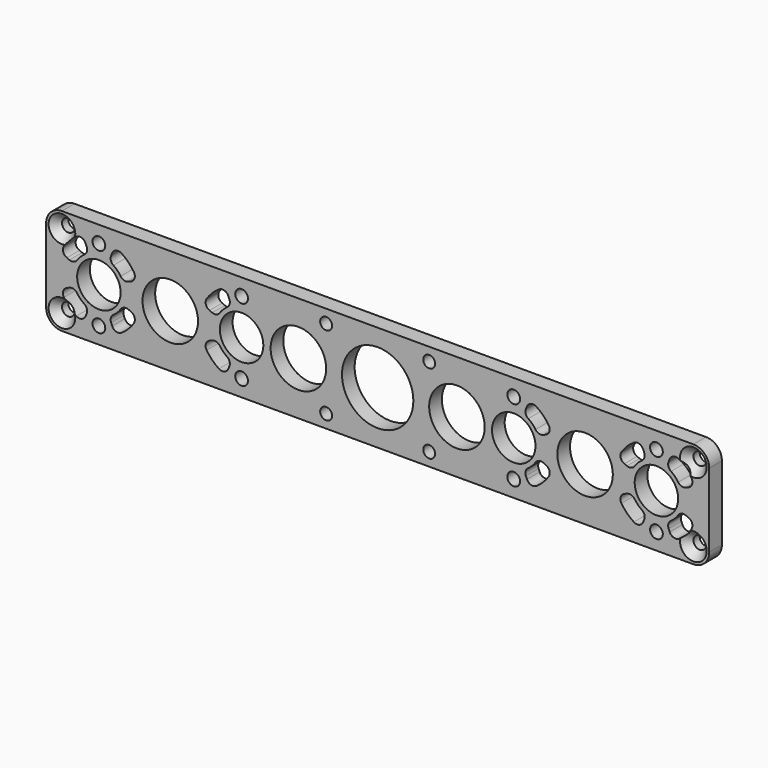
from build123d import *

# Parameters (mm, degrees)
F0_R      = 2.5527
F0_R_2    = 8.6995
F0_R_3    = 11.1125
F0_R_4    = 14.2875
F1_DEPTH  = 6.35
F2_R      = 2.38125
F3_DEPTH  = 6.351
F15_DEPTH = 25.4


with BuildPart() as f1:
    # F0 (on Front) → F1 (new body)
    with BuildSketch(Plane.XZ):
        with BuildLine():
            Line((111.633, 21.1455), (-111.633, 21.1455))
            Line((-111.633, 21.1455), (-126.4285, 21.1455))
            ThreePointArc((-126.4285, 21.1455), (-130.9186280605, 19.2856280605), (-132.7785, 14.7955))
            Line((-132.7785, 14.7955), (-132.7785, -14.7955))
            ThreePointArc((-132.7785, -14.7955), (-130.9186280605, -19.2856280605), (-126.4285, -21.1455))
            Line((-126.4285, -21.1455), (-111.633, -21.1455))
            Line((-111.633, -21.1455), (111.633, -21.1455))
            Line((111.633, -21.1455), (126.4285, -21.1455))
            ThreePointArc((126.4285, -21.1455), (130.9186280605, -19.2856280605), (132.7785, -14.7955))
            Line((132.7785, -14.7955), (132.7785, 14.7955))
            ThreePointArc((132.7785, 14.7955), (130.9186280605, 19.2856280605), (126.4285, 21.1455))
            Line((126.4285, 21.1455), (111.633, 21.1455))
        make_face()
        with Locations((-126.4285, -14.7955)):
            Circle(F0_R, mode=Mode.SUBTRACT)
        with Locations((-111.633, -14.5)):
            Circle(F0_R, mode=Mode.SUBTRACT)
        with Locations((-54.483, -14.5)):
            Circle(F0_R, mode=Mode.SUBTRACT)
        with Locations((54.483, -14.5)):
            Circle(F0_R, mode=Mode.SUBTRACT)
        with Locations((111.633, -14.5)):
            Circle(F0_R, mode=Mode.SUBTRACT)
        with Locations((126.4285, -14.7955)):
            Circle(F0_R, mode=Mode.SUBTRACT)
        with Locations((-111.633, 0)):
            Circle(F0_R_2, mode=Mode.SUBTRACT)
        with Locations((-83.058, 0)):
            Circle(F0_R_3, mode=Mode.SUBTRACT)
        with Locations((-54.483, 0)):
            Circle(F0_R_2, mode=Mode.SUBTRACT)
        with Locations((-31.75, 0)):
            Circle(F0_R_3, mode=Mode.SUBTRACT)
        with Locations((-126.4285, 14.7955)):
            Circle(F0_R, mode=Mode.SUBTRACT)
        with Locations((-111.633, 14.5)):
            Circle(F0_R, mode=Mode.SUBTRACT)
        with Locations((-54.483, 14.5)):
            Circle(F0_R, mode=Mode.SUBTRACT)
        Circle(F0_R_4, mode=Mode.SUBTRACT)
        with Locations((31.75, 0)):
            Circle(F0_R_3, mode=Mode.SUBTRACT)
        with Locations((54.483, 0)):
            Circle(F0_R_2, mode=Mode.SUBTRACT)
        with Locations((83.058, 0)):
            Circle(F0_R_3, mode=Mode.SUBTRACT)
        with Locations((111.633, 0)):
            Circle(F0_R_2, mode=Mode.SUBTRACT)
        with Locations((54.483, 14.5)):
            Circle(F0_R, mode=Mode.SUBTRACT)
        with Locations((111.633, 14.5)):
            Circle(F0_R, mode=Mode.SUBTRACT)
        with Locations((126.4285, 14.7955)):
            Circle(F0_R, mode=Mode.SUBTRACT)
    extrude(amount=F1_DEPTH)

    # F2 (on face) → F3 (cut, through all)
    with BuildSketch(Plane.XZ.offset(6.35)):
        with Locations((20.6375, 15.875)):
            Circle(F2_R)
        with Locations((20.6375, -15.875)):
            Circle(F2_R)
        with Locations((-20.6375, -15.875)):
            Circle(F2_R)
        with Locations((-20.6375, 15.875)):
            Circle(F2_R)
    extrude(amount=-F3_DEPTH, mode=Mode.SUBTRACT)

    # F5 (on offset) → F6 (revolve, cut)
    with BuildSketch(Plane.YZ.offset(126.4285)):
        Polygon((-6.35, 20.1396451588), (-6.35, 14.7955), (-3.1242, 14.7955), (-3.1242, 17.3355), align=None)
    revolve(axis=Axis((126.4285, -4.7371, 14.7955), (0, 1, 0)), mode=Mode.SUBTRACT)

    # F7 (on offset) → F8 (revolve, cut)
    with BuildSketch(Plane.YZ.offset(126.4285)):
        Polygon((-6.35, -9.4513548412), (-6.35, -14.7955), (-3.1242, -14.7955), (-3.1242, -12.2555), align=None)
    revolve(axis=Axis((126.4285, -4.7371, -14.7955), (0, 1, 0)), mode=Mode.SUBTRACT)

    # F10 (on offset) → F11 (revolve, cut)
    with BuildSketch(Plane(origin=(-126.4285, 0, 0), x_dir=(0, -1, 0), z_dir=(-1, 0, 0))):
        Polygon((6.35, 9.4513548412), (6.35, 14.7955), (3.1242, 14.7955), (3.1242, 12.2555), align=None)
    revolve(axis=Axis((-126.4285, -4.7371, 14.7955), (0, 1, 0)), mode=Mode.SUBTRACT)

    # F12 (on offset) → F13 (revolve, cut)
    with BuildSketch(Plane(origin=(-126.4285, 0, 0), x_dir=(0, -1, 0), z_dir=(-1, 0, 0))):
        Polygon((6.35, -20.1396451588), (6.35, -14.7955), (3.1242, -14.7955), (3.1242, -17.3355), align=None)
    revolve(axis=Axis((-126.4285, -4.7371, -14.7955), (0, 1, 0)), mode=Mode.SUBTRACT)

    # F14 (on face) → F15 (cut)
    with BuildSketch(Plane(origin=(0, 0, 0), x_dir=(-1, 0, 0), z_dir=(0, 1, 0))):
        with BuildLine():
            Line((106.3142512649, -12.840595331), (106.7471694564, -11.7954383619))
            ThreePointArc((106.7471694564, -11.7954383619), (106.8311557852, -10.0861385562), (105.8117319426, -8.7115351376))
            ThreePointArc((105.8117319426, -8.7115351376), (104.2242887001, -7.4087112999), (102.9214648624, -5.8212680574))
            ThreePointArc((102.9214648624, -5.8212680574), (101.5468614438, -4.8018442148), (99.8375616381, -4.8858305436))
            Line((99.8375616381, -4.8858305436), (98.792404669, -5.3187487351))
            ThreePointArc((98.792404669, -5.3187487351), (97.3396139347, -6.9091536496), (97.6307433893, -9.0434526798))
            ThreePointArc((97.6307433893, -9.0434526798), (99.8464138411, -11.7865861589), (102.5895473202, -14.0022566107))
            ThreePointArc((102.5895473202, -14.0022566107), (104.7238463504, -14.2933860653), (106.3142512649, -12.840595331))
        make_face()
        with BuildLine():
            Line((98.792404669, 5.3187487351), (99.8375616381, 4.8858305436))
            ThreePointArc((99.8375616381, 4.8858305436), (101.5468614438, 4.8018442148), (102.9214648624, 5.8212680574))
            ThreePointArc((102.9214648624, 5.8212680574), (104.2242887001, 7.4087112999), (105.8117319426, 8.7115351376))
            ThreePointArc((105.8117319426, 8.7115351376), (106.8311557852, 10.0861385562), (106.7471694564, 11.7954383619))
            Line((106.7471694564, 11.7954383619), (106.3142512649, 12.840595331))
            ThreePointArc((106.3142512649, 12.840595331), (104.7238463504, 14.2933860653), (102.5895473202, 14.0022566107))
            ThreePointArc((102.5895473202, 14.0022566107), (99.8464138411, 11.7865861589), (97.6307433893, 9.0434526798))
            ThreePointArc((97.6307433893, 9.0434526798), (97.3396139347, 6.9091536496), (98.792404669, 5.3187487351))
        make_face()
        with BuildLine():
            Line((116.9517487351, 12.840595331), (116.5188305436, 11.7954383619))
            ThreePointArc((116.5188305436, 11.7954383619), (116.4348442148, 10.0861385562), (117.4542680574, 8.7115351376))
            ThreePointArc((117.4542680574, 8.7115351376), (119.0417112999, 7.4087112999), (120.3445351376, 5.8212680574))
            ThreePointArc((120.3445351376, 5.8212680574), (121.7191385562, 4.8018442148), (123.4284383619, 4.8858305436))
            Line((123.4284383619, 4.8858305436), (124.473595331, 5.3187487351))
            ThreePointArc((124.473595331, 5.3187487351), (125.9263860653, 6.9091536496), (125.6352566107, 9.0434526798))
            ThreePointArc((125.6352566107, 9.0434526798), (123.4195861589, 11.7865861589), (120.6764526798, 14.0022566107))
            ThreePointArc((120.6764526798, 14.0022566107), (118.5421536496, 14.2933860653), (116.9517487351, 12.840595331))
        make_face()
        with BuildLine():
            Line((124.473595331, -5.3187487351), (123.4284383619, -4.8858305436))
            ThreePointArc((123.4284383619, -4.8858305436), (121.7191385562, -4.8018442148), (120.3445351376, -5.8212680574))
            ThreePointArc((120.3445351376, -5.8212680574), (119.0417112999, -7.4087112999), (117.4542680574, -8.7115351376))
            ThreePointArc((117.4542680574, -8.7115351376), (116.4348442148, -10.0861385562), (116.5188305436, -11.7954383619))
            Line((116.5188305436, -11.7954383619), (116.9517487351, -12.840595331))
            ThreePointArc((116.9517487351, -12.840595331), (118.5421536496, -14.2933860653), (120.6764526798, -14.0022566107))
            ThreePointArc((120.6764526798, -14.0022566107), (123.4195861589, -11.7865861589), (125.6352566107, -9.0434526798))
            ThreePointArc((125.6352566107, -9.0434526798), (125.9263860653, -6.9091536496), (124.473595331, -5.3187487351))
        make_face()
        with BuildLine():
            Line((59.8017487351, 12.840595331), (59.3688305436, 11.7954383619))
            ThreePointArc((59.3688305436, 11.7954383619), (59.2848442148, 10.0861385562), (60.3042680574, 8.7115351376))
            ThreePointArc((60.3042680574, 8.7115351376), (61.8917112999, 7.4087112999), (63.1945351376, 5.8212680574))
            ThreePointArc((63.1945351376, 5.8212680574), (64.5691385562, 4.8018442148), (66.2784383619, 4.8858305436))
            Line((66.2784383619, 4.8858305436), (67.323595331, 5.3187487351))
            ThreePointArc((67.323595331, 5.3187487351), (68.7763860653, 6.9091536496), (68.4852566107, 9.0434526798))
            ThreePointArc((68.4852566107, 9.0434526798), (66.2695861589, 11.7865861589), (63.5264526798, 14.0022566107))
            ThreePointArc((63.5264526798, 14.0022566107), (61.3921536496, 14.2933860653), (59.8017487351, 12.840595331))
        make_face()
        with BuildLine():
            Line((67.323595331, -5.3187487351), (66.2784383619, -4.8858305436))
            ThreePointArc((66.2784383619, -4.8858305436), (64.5691385562, -4.8018442148), (63.1945351376, -5.8212680574))
            ThreePointArc((63.1945351376, -5.8212680574), (61.8917112999, -7.4087112999), (60.3042680574, -8.7115351376))
            ThreePointArc((60.3042680574, -8.7115351376), (59.2848442148, -10.0861385562), (59.3688305436, -11.7954383619))
            Line((59.3688305436, -11.7954383619), (59.8017487351, -12.840595331))
            ThreePointArc((59.8017487351, -12.840595331), (61.3921536496, -14.2933860653), (63.5264526798, -14.0022566107))
            ThreePointArc((63.5264526798, -14.0022566107), (66.2695861589, -11.7865861589), (68.4852566107, -9.0434526798))
            ThreePointArc((68.4852566107, -9.0434526798), (68.7763860653, -6.9091536496), (67.323595331, -5.3187487351))
        make_face()
        with BuildLine():
            Line((-59.8017487351, -12.840595331), (-59.3688305436, -11.7954383619))
            ThreePointArc((-59.3688305436, -11.7954383619), (-59.2848442148, -10.0861385562), (-60.3042680574, -8.7115351376))
            ThreePointArc((-60.3042680574, -8.7115351376), (-61.8917112999, -7.4087112999), (-63.1945351376, -5.8212680574))
            ThreePointArc((-63.1945351376, -5.8212680574), (-64.5691385562, -4.8018442148), (-66.2784383619, -4.8858305436))
            Line((-66.2784383619, -4.8858305436), (-67.323595331, -5.3187487351))
            ThreePointArc((-67.323595331, -5.3187487351), (-68.7763860653, -6.9091536496), (-68.4852566107, -9.0434526798))
            ThreePointArc((-68.4852566107, -9.0434526798), (-66.2695861589, -11.7865861589), (-63.5264526798, -14.0022566107))
            ThreePointArc((-63.5264526798, -14.0022566107), (-61.3921536496, -14.2933860653), (-59.8017487351, -12.840595331))
        make_face()
        with BuildLine():
            Line((-67.323595331, 5.3187487351), (-66.2784383619, 4.8858305436))
            ThreePointArc((-66.2784383619, 4.8858305436), (-64.5691385562, 4.8018442148), (-63.1945351376, 5.8212680574))
            ThreePointArc((-63.1945351376, 5.8212680574), (-61.8917112999, 7.4087112999), (-60.3042680574, 8.7115351376))
            ThreePointArc((-60.3042680574, 8.7115351376), (-59.2848442148, 10.0861385562), (-59.3688305436, 11.7954383619))
            Line((-59.3688305436, 11.7954383619), (-59.8017487351, 12.840595331))
            ThreePointArc((-59.8017487351, 12.840595331), (-61.3921536496, 14.2933860653), (-63.5264526798, 14.0022566107))
            ThreePointArc((-63.5264526798, 14.0022566107), (-66.2695861589, 11.7865861589), (-68.4852566107, 9.0434526798))
            ThreePointArc((-68.4852566107, 9.0434526798), (-68.7763860653, 6.9091536496), (-67.323595331, 5.3187487351))
        make_face()
        with BuildLine():
            Line((-116.9517487351, -12.840595331), (-116.5188305436, -11.7954383619))
            ThreePointArc((-116.5188305436, -11.7954383619), (-116.4348442148, -10.0861385562), (-117.4542680574, -8.7115351376))
            ThreePointArc((-117.4542680574, -8.7115351376), (-119.0417112999, -7.4087112999), (-120.3445351376, -5.8212680574))
            ThreePointArc((-120.3445351376, -5.8212680574), (-121.7191385562, -4.8018442148), (-123.4284383619, -4.8858305436))
            Line((-123.4284383619, -4.8858305436), (-124.473595331, -5.3187487351))
            ThreePointArc((-124.473595331, -5.3187487351), (-125.9263860653, -6.9091536496), (-125.6352566107, -9.0434526798))
            ThreePointArc((-125.6352566107, -9.0434526798), (-123.4195861589, -11.7865861589), (-120.6764526798, -14.0022566107))
            ThreePointArc((-120.6764526798, -14.0022566107), (-118.5421536496, -14.2933860653), (-116.9517487351, -12.840595331))
        make_face()
        with BuildLine():
            Line((-124.473595331, 5.3187487351), (-123.4284383619, 4.8858305436))
            ThreePointArc((-123.4284383619, 4.8858305436), (-121.7191385562, 4.8018442148), (-120.3445351376, 5.8212680574))
            ThreePointArc((-120.3445351376, 5.8212680574), (-119.0417112999, 7.4087112999), (-117.4542680574, 8.7115351376))
            ThreePointArc((-117.4542680574, 8.7115351376), (-116.4348442148, 10.0861385562), (-116.5188305436, 11.7954383619))
            Line((-116.5188305436, 11.7954383619), (-116.9517487351, 12.840595331))
            ThreePointArc((-116.9517487351, 12.840595331), (-118.5421536496, 14.2933860653), (-120.6764526798, 14.0022566107))
            ThreePointArc((-120.6764526798, 14.0022566107), (-123.4195861589, 11.7865861589), (-125.6352566107, 9.0434526798))
            ThreePointArc((-125.6352566107, 9.0434526798), (-125.9263860653, 6.9091536496), (-124.473595331, 5.3187487351))
        make_face()
        with BuildLine():
            Line((-106.3142512649, 12.840595331), (-106.7471694564, 11.7954383619))
            ThreePointArc((-106.7471694564, 11.7954383619), (-106.8311557852, 10.0861385562), (-105.8117319426, 8.7115351376))
            ThreePointArc((-105.8117319426, 8.7115351376), (-104.2242887001, 7.4087112999), (-102.9214648624, 5.8212680574))
            ThreePointArc((-102.9214648624, 5.8212680574), (-101.5468614438, 4.8018442148), (-99.8375616381, 4.8858305436))
            Line((-99.8375616381, 4.8858305436), (-98.792404669, 5.3187487351))
            ThreePointArc((-98.792404669, 5.3187487351), (-97.3396139347, 6.9091536496), (-97.6307433893, 9.0434526798))
            ThreePointArc((-97.6307433893, 9.0434526798), (-99.8464138411, 11.7865861589), (-102.5895473202, 14.0022566107))
            ThreePointArc((-102.5895473202, 14.0022566107), (-104.7238463504, 14.2933860653), (-106.3142512649, 12.840595331))
        make_face()
        with BuildLine():
            Line((-98.792404669, -5.3187487351), (-99.8375616381, -4.8858305436))
            ThreePointArc((-99.8375616381, -4.8858305436), (-101.5468614438, -4.8018442148), (-102.9214648624, -5.8212680574))
            ThreePointArc((-102.9214648624, -5.8212680574), (-104.2242887001, -7.4087112999), (-105.8117319426, -8.7115351376))
            ThreePointArc((-105.8117319426, -8.7115351376), (-106.8311557852, -10.0861385562), (-106.7471694564, -11.7954383619))
            Line((-106.7471694564, -11.7954383619), (-106.3142512649, -12.840595331))
            ThreePointArc((-106.3142512649, -12.840595331), (-104.7238463504, -14.2933860653), (-102.5895473202, -14.0022566107))
            ThreePointArc((-102.5895473202, -14.0022566107), (-99.8464138411, -11.7865861589), (-97.6307433893, -9.0434526798))
            ThreePointArc((-97.6307433893, -9.0434526798), (-97.3396139347, -6.9091536496), (-98.792404669, -5.3187487351))
        make_face()
    extrude(amount=-F15_DEPTH, mode=Mode.SUBTRACT)


solid = f1.part
